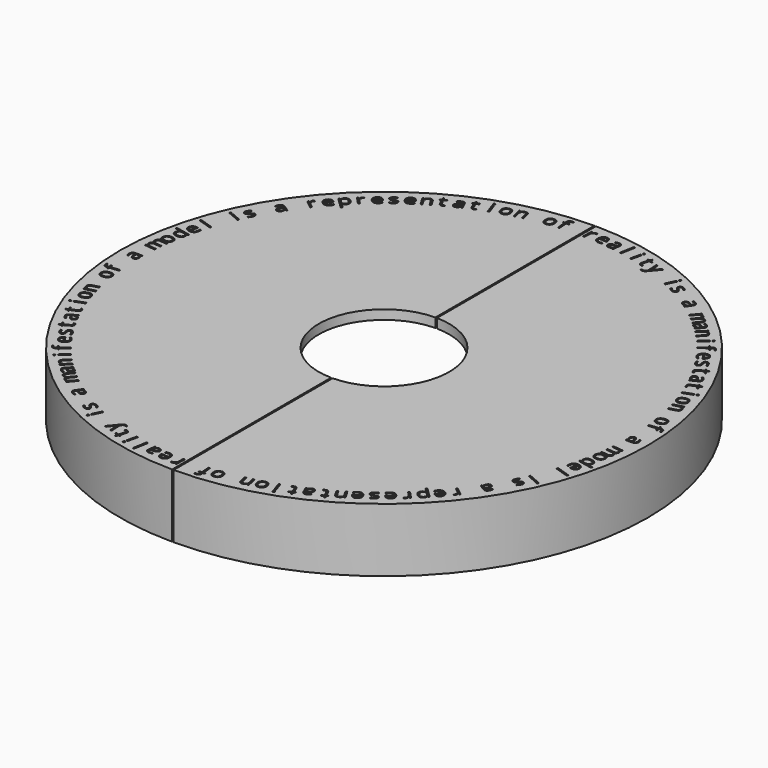
from build123d import *

# Parameters (mm, degrees)
F3_TEXT_SIZE = 6.25
F4_DEPTH     = 0.5
F5_W         = 0.5
F5_H         = 250
F6_DEPTH     = 20.5010001
F7_R         = 1.5
F8_DEPTH     = 1.5


# Not quite as in the source:
# - Text() gives the source's letters only with a copy of the font that has no kerning and outlines rounded to 1/6400 em; it was checked with that copy


with BuildPart() as f1:
    # F0 (on Front) → F1 (revolve)
    with BuildSketch(Plane.XZ):
        Polygon((-80.75, 17.5), (-21, 17.5), (-21, 20.5), (-80.75, 20.5), (-85, 20.5), (-85, 0), (-80.75, 0), align=None)
    revolve(axis=Axis((0, 0, 4.5), (0, 0, 1)))

    # F3 (on face) → F4 (cut)
    with BuildSketch(Plane.XY.offset(20.5)):
        with Locations(Location((78.75, 1.6875), (0, 0, -90))):
            Text('a', F3_TEXT_SIZE, font='Open Sans', text_align=(TextAlign.LEFT, TextAlign.BOTTOM))
        with Locations(Location((78.6262675544, -5.2563334208), (0, 0, -95.9016393443))):
            Text('m', F3_TEXT_SIZE, font='Open Sans', text_align=(TextAlign.LEFT, TextAlign.BOTTOM))
        with Locations(Location((78.106553141, -10.227138462), (0, 0, -98.8524590164))):
            Text('o', F3_TEXT_SIZE, font='Open Sans', text_align=(TextAlign.LEFT, TextAlign.BOTTOM))
        with Locations(Location((77.4631267415, -14.2984525124), (0, 0, -101.8032786885))):
            Text('d', F3_TEXT_SIZE, font='Open Sans', text_align=(TextAlign.LEFT, TextAlign.BOTTOM))
        with Locations(Location((76.6099263363, -18.3219724096), (0, 0, -104.7540983607))):
            Text('e', F3_TEXT_SIZE, font='Open Sans', text_align=(TextAlign.LEFT, TextAlign.BOTTOM))
        with Locations(Location((75.2404006968, -23.2587545179), (0, 0, -107.7049180328))):
            Text('l', F3_TEXT_SIZE, font='Open Sans', text_align=(TextAlign.LEFT, TextAlign.BOTTOM))
        with Locations(Location((72.4599055893, -30.8494022324), (0, 0, -113.606557377))):
            Text('i', F3_TEXT_SIZE, font='Open Sans', text_align=(TextAlign.LEFT, TextAlign.BOTTOM))
        with Locations(Location((71.1337657816, -33.8223559246), (0, 0, -116.5573770492))):
            Text('s', F3_TEXT_SIZE, font='Open Sans', text_align=(TextAlign.LEFT, TextAlign.BOTTOM))
        with Locations(Location((67.3530001634, -40.8409540196), (0, 0, -122.4590163934))):
            Text('a', F3_TEXT_SIZE, font='Open Sans', text_align=(TextAlign.LEFT, TextAlign.BOTTOM))
        with Locations(Location((12.0100738883, -77.8523354171), (0, 0, -172.6229508197))):
            Text('o', F3_TEXT_SIZE, font='Open Sans', text_align=(TextAlign.LEFT, TextAlign.BOTTOM))
        with Locations(Location((57.7536819392, -53.5710114351), (0, 0, -134.262295082))):
            Text('p', F3_TEXT_SIZE, font='Open Sans', text_align=(TextAlign.LEFT, TextAlign.BOTTOM))
        with Locations(Location((62.6394396742, -47.748504569), (0, 0, -128.3606557377))):
            Text('r', F3_TEXT_SIZE, font='Open Sans', text_align=(TextAlign.LEFT, TextAlign.BOTTOM))
        with Locations(Location((60.3349493388, -50.6405901873), (0, 0, -131.3114754098))):
            Text('e', F3_TEXT_SIZE, font='Open Sans', text_align=(TextAlign.LEFT, TextAlign.BOTTOM))
        with Locations(Location((54.5452272552, -56.8193389169), (0, 0, -137.2131147541))):
            Text('r', F3_TEXT_SIZE, font='Open Sans', text_align=(TextAlign.LEFT, TextAlign.BOTTOM))
        with Locations(Location((51.8231235243, -59.3223343642), (0, 0, -140.1639344262))):
            Text('e', F3_TEXT_SIZE, font='Open Sans', text_align=(TextAlign.LEFT, TextAlign.BOTTOM))
        with Locations(Location((48.5064692039, -62.0571256178), (0, 0, -143.1147540984))):
            Text('s', F3_TEXT_SIZE, font='Open Sans', text_align=(TextAlign.LEFT, TextAlign.BOTTOM))
        with Locations(Location((42.1423747186, -66.5513068223), (0, 0, -149.0163934426))):
            Text('n', F3_TEXT_SIZE, font='Open Sans', text_align=(TextAlign.LEFT, TextAlign.BOTTOM))
        with Locations(Location((45.4488729518, -64.3364238487), (0, 0, -146.0655737705))):
            Text('e', F3_TEXT_SIZE, font='Open Sans', text_align=(TextAlign.LEFT, TextAlign.BOTTOM))
        with Locations(Location((38.1053971012, -68.928074056), (0, 0, -151.9672131148))):
            Text('t', F3_TEXT_SIZE, font='Open Sans', text_align=(TextAlign.LEFT, TextAlign.BOTTOM))
        with Locations(Location((34.9116308373, -70.6086976833), (0, 0, -154.9180327869))):
            Text('a', F3_TEXT_SIZE, font='Open Sans', text_align=(TextAlign.LEFT, TextAlign.BOTTOM))
        with Locations(Location((30.8161804516, -72.4807816161), (0, 0, -157.868852459))):
            Text('t', F3_TEXT_SIZE, font='Open Sans', text_align=(TextAlign.LEFT, TextAlign.BOTTOM))
        with Locations(Location((26.5801571443, -74.1324408225), (0, 0, -160.8196721311))):
            Text('i', F3_TEXT_SIZE, font='Open Sans', text_align=(TextAlign.LEFT, TextAlign.BOTTOM))
        with Locations(Location((23.8477494353, -75.0767131111), (0, 0, -163.7704918033))):
            Text('o', F3_TEXT_SIZE, font='Open Sans', text_align=(TextAlign.LEFT, TextAlign.BOTTOM))
        with Locations(Location((7.4694002148, -78.4073935642), (0, 0, -175.5737704918))):
            Text('f', F3_TEXT_SIZE, font='Open Sans', text_align=(TextAlign.LEFT, TextAlign.BOTTOM))
        with Locations(Location((19.9070776726, -76.215250739), (0, 0, -166.7213114754))):
            Text('n', F3_TEXT_SIZE, font='Open Sans', text_align=(TextAlign.LEFT, TextAlign.BOTTOM))
        with Locations(Location((-0.5940416139, -78.7608164371), (0, 0, 178.5245901639))):
            Text('r', F3_TEXT_SIZE, font='Open Sans', text_align=(TextAlign.LEFT, TextAlign.BOTTOM))
        with Locations(Location((-4.2904331993, -78.6534657164), (0, 0, 175.5737704918))):
            Text('e', F3_TEXT_SIZE, font='Open Sans', text_align=(TextAlign.LEFT, TextAlign.BOTTOM))
        with Locations(Location((-8.4378384552, -78.3148328125), (0, 0, 172.6229508197))):
            Text('a', F3_TEXT_SIZE, font='Open Sans', text_align=(TextAlign.LEFT, TextAlign.BOTTOM))
        with Locations(Location((-13.4054905375, -77.603997205), (0, 0, 169.6721311475))):
            Text('l', F3_TEXT_SIZE, font='Open Sans', text_align=(TextAlign.LEFT, TextAlign.BOTTOM))
        with Locations(Location((-17.3589118661, -76.8166109311), (0, 0, 166.7213114754))):
            Text('i', F3_TEXT_SIZE, font='Open Sans', text_align=(TextAlign.LEFT, TextAlign.BOTTOM))
        with Locations(Location((-20.8186828661, -75.9584302433), (0, 0, 163.7704918033))):
            Text('t', F3_TEXT_SIZE, font='Open Sans', text_align=(TextAlign.LEFT, TextAlign.BOTTOM))
        with Locations(Location((-24.196797606, -74.9614969893), (0, 0, 160.8196721311))):
            Text('y', F3_TEXT_SIZE, font='Open Sans', text_align=(TextAlign.LEFT, TextAlign.BOTTOM))
        with Locations(Location((-32.704866046, -71.6415750317), (0, 0, 154.9180327869))):
            Text('i', F3_TEXT_SIZE, font='Open Sans', text_align=(TextAlign.LEFT, TextAlign.BOTTOM))
        with Locations(Location((-35.6426887742, -70.2393275275), (0, 0, 151.9672131148))):
            Text('s', F3_TEXT_SIZE, font='Open Sans', text_align=(TextAlign.LEFT, TextAlign.BOTTOM))
        with Locations(Location((-42.5616131492, -66.2791010982), (0, 0, 146.0655737705))):
            Text('a', F3_TEXT_SIZE, font='Open Sans', text_align=(TextAlign.LEFT, TextAlign.BOTTOM))
        with Locations(Location((-48.2536792635, -62.3000917183), (0, 0, 140.1639344262))):
            Text('m', F3_TEXT_SIZE, font='Open Sans', text_align=(TextAlign.LEFT, TextAlign.BOTTOM))
        with Locations(Location((-52.2543438823, -58.9397463659), (0, 0, 137.2131147541))):
            Text('a', F3_TEXT_SIZE, font='Open Sans', text_align=(TextAlign.LEFT, TextAlign.BOTTOM))
        with Locations(Location((-55.0924290561, -56.3016913367), (0, 0, 134.262295082))):
            Text('n', F3_TEXT_SIZE, font='Open Sans', text_align=(TextAlign.LEFT, TextAlign.BOTTOM))
        with Locations(Location((-58.6571701454, -52.5495949237), (0, 0, 131.3114754098))):
            Text('i', F3_TEXT_SIZE, font='Open Sans', text_align=(TextAlign.LEFT, TextAlign.BOTTOM))
        with Locations(Location((-60.8830663555, -49.9676248809), (0, 0, 128.3606557377))):
            Text('f', F3_TEXT_SIZE, font='Open Sans', text_align=(TextAlign.LEFT, TextAlign.BOTTOM))
        with Locations(Location((-63.1448805777, -47.0903338601), (0, 0, 125.4098360656))):
            Text('e', F3_TEXT_SIZE, font='Open Sans', text_align=(TextAlign.LEFT, TextAlign.BOTTOM))
        with Locations(Location((-65.6155510589, -43.5725125947), (0, 0, 122.4590163934))):
            Text('s', F3_TEXT_SIZE, font='Open Sans', text_align=(TextAlign.LEFT, TextAlign.BOTTOM))
        with Locations(Location((-67.9240876859, -39.8675180233), (0, 0, 119.5081967213))):
            Text('t', F3_TEXT_SIZE, font='Open Sans', text_align=(TextAlign.LEFT, TextAlign.BOTTOM))
        with Locations(Location((-69.6863869499, -36.7180831488), (0, 0, 116.5573770492))):
            Text('a', F3_TEXT_SIZE, font='Open Sans', text_align=(TextAlign.LEFT, TextAlign.BOTTOM))
        with Locations(Location((-71.663299529, -32.6721927934), (0, 0, 113.606557377))):
            Text('t', F3_TEXT_SIZE, font='Open Sans', text_align=(TextAlign.LEFT, TextAlign.BOTTOM))
        with Locations(Location((-73.423479919, -28.4801006441), (0, 0, 110.6557377049))):
            Text('i', F3_TEXT_SIZE, font='Open Sans', text_align=(TextAlign.LEFT, TextAlign.BOTTOM))
        with Locations(Location((-74.4377929484, -25.7729118584), (0, 0, 107.7049180328))):
            Text('o', F3_TEXT_SIZE, font='Open Sans', text_align=(TextAlign.LEFT, TextAlign.BOTTOM))
        with Locations(Location((-75.6774171905, -21.8628615249), (0, 0, 104.7540983607))):
            Text('n', F3_TEXT_SIZE, font='Open Sans', text_align=(TextAlign.LEFT, TextAlign.BOTTOM))
        with Locations(Location((-77.5172904933, -14.0106273688), (0, 0, 98.8524590164))):
            Text('o', F3_TEXT_SIZE, font='Open Sans', text_align=(TextAlign.LEFT, TextAlign.BOTTOM))
        with Locations(Location((-78.1890774943, -9.4857506654), (0, 0, 95.9016393443))):
            Text('f', F3_TEXT_SIZE, font='Open Sans', text_align=(TextAlign.LEFT, TextAlign.BOTTOM))
        with Locations(Location((-78.75, -1.6875), (0, 0, 90))):
            Text('a', F3_TEXT_SIZE, font='Open Sans', text_align=(TextAlign.LEFT, TextAlign.BOTTOM))
        with Locations(Location((-78.6262675544, 5.2563334208), (0, 0, 84.0983606557))):
            Text('m', F3_TEXT_SIZE, font='Open Sans', text_align=(TextAlign.LEFT, TextAlign.BOTTOM))
        with Locations(Location((-78.106553141, 10.227138462), (0, 0, 81.1475409836))):
            Text('o', F3_TEXT_SIZE, font='Open Sans', text_align=(TextAlign.LEFT, TextAlign.BOTTOM))
        with Locations(Location((-77.4631267415, 14.2984525124), (0, 0, 78.1967213115))):
            Text('d', F3_TEXT_SIZE, font='Open Sans', text_align=(TextAlign.LEFT, TextAlign.BOTTOM))
        with Locations(Location((-76.6099263363, 18.3219724096), (0, 0, 75.2459016393))):
            Text('e', F3_TEXT_SIZE, font='Open Sans', text_align=(TextAlign.LEFT, TextAlign.BOTTOM))
        with Locations(Location((-75.2404006968, 23.2587545179), (0, 0, 72.2950819672))):
            Text('l', F3_TEXT_SIZE, font='Open Sans', text_align=(TextAlign.LEFT, TextAlign.BOTTOM))
        with Locations(Location((-72.4599055893, 30.8494022324), (0, 0, 66.393442623))):
            Text('i', F3_TEXT_SIZE, font='Open Sans', text_align=(TextAlign.LEFT, TextAlign.BOTTOM))
        with Locations(Location((-71.1337657816, 33.8223559246), (0, 0, 63.4426229508))):
            Text('s', F3_TEXT_SIZE, font='Open Sans', text_align=(TextAlign.LEFT, TextAlign.BOTTOM))
        with Locations(Location((-67.3530001634, 40.8409540196), (0, 0, 57.5409836066))):
            Text('a', F3_TEXT_SIZE, font='Open Sans', text_align=(TextAlign.LEFT, TextAlign.BOTTOM))
        with Locations(Location((-62.6394396742, 47.748504569), (0, 0, 51.6393442623))):
            Text('r', F3_TEXT_SIZE, font='Open Sans', text_align=(TextAlign.LEFT, TextAlign.BOTTOM))
        with Locations(Location((-60.3349493388, 50.6405901873), (0, 0, 48.6885245902))):
            Text('e', F3_TEXT_SIZE, font='Open Sans', text_align=(TextAlign.LEFT, TextAlign.BOTTOM))
        with Locations(Location((-57.7536819392, 53.5710114351), (0, 0, 45.737704918))):
            Text('p', F3_TEXT_SIZE, font='Open Sans', text_align=(TextAlign.LEFT, TextAlign.BOTTOM))
        with Locations(Location((-54.5452272552, 56.8193389169), (0, 0, 42.7868852459))):
            Text('r', F3_TEXT_SIZE, font='Open Sans', text_align=(TextAlign.LEFT, TextAlign.BOTTOM))
        with Locations(Location((-51.8231235243, 59.3223343642), (0, 0, 39.8360655738))):
            Text('e', F3_TEXT_SIZE, font='Open Sans', text_align=(TextAlign.LEFT, TextAlign.BOTTOM))
        with Locations(Location((-48.5064692039, 62.0571256178), (0, 0, 36.8852459016))):
            Text('s', F3_TEXT_SIZE, font='Open Sans', text_align=(TextAlign.LEFT, TextAlign.BOTTOM))
        with Locations(Location((-45.4488729518, 64.3364238487), (0, 0, 33.9344262295))):
            Text('e', F3_TEXT_SIZE, font='Open Sans', text_align=(TextAlign.LEFT, TextAlign.BOTTOM))
        with Locations(Location((-42.1423747186, 66.5513068223), (0, 0, 30.9836065574))):
            Text('n', F3_TEXT_SIZE, font='Open Sans', text_align=(TextAlign.LEFT, TextAlign.BOTTOM))
        with Locations(Location((-38.1053971012, 68.928074056), (0, 0, 28.0327868852))):
            Text('t', F3_TEXT_SIZE, font='Open Sans', text_align=(TextAlign.LEFT, TextAlign.BOTTOM))
        with Locations(Location((-34.9116308373, 70.6086976833), (0, 0, 25.0819672131))):
            Text('a', F3_TEXT_SIZE, font='Open Sans', text_align=(TextAlign.LEFT, TextAlign.BOTTOM))
        with Locations(Location((-30.8161804516, 72.4807816161), (0, 0, 22.131147541))):
            Text('t', F3_TEXT_SIZE, font='Open Sans', text_align=(TextAlign.LEFT, TextAlign.BOTTOM))
        with Locations(Location((-26.5801571443, 74.1324408225), (0, 0, 19.1803278689))):
            Text('i', F3_TEXT_SIZE, font='Open Sans', text_align=(TextAlign.LEFT, TextAlign.BOTTOM))
        with Locations(Location((-23.8477494353, 75.0767131111), (0, 0, 16.2295081967))):
            Text('o', F3_TEXT_SIZE, font='Open Sans', text_align=(TextAlign.LEFT, TextAlign.BOTTOM))
        with Locations(Location((-19.9070776726, 76.215250739), (0, 0, 13.2786885246))):
            Text('n', F3_TEXT_SIZE, font='Open Sans', text_align=(TextAlign.LEFT, TextAlign.BOTTOM))
        with Locations(Location((-12.0100738883, 77.8523354171), (0, 0, 7.3770491803))):
            Text('o', F3_TEXT_SIZE, font='Open Sans', text_align=(TextAlign.LEFT, TextAlign.BOTTOM))
        with Locations(Location((-7.4694002148, 78.4073935642), (0, 0, 4.4262295082))):
            Text('f', F3_TEXT_SIZE, font='Open Sans', text_align=(TextAlign.LEFT, TextAlign.BOTTOM))
        with Locations(Location((0.5940416139, 78.7608164371), (0, 0, -1.4754098361))):
            Text('r', F3_TEXT_SIZE, font='Open Sans', text_align=(TextAlign.LEFT, TextAlign.BOTTOM))
        with Locations(Location((4.2904331993, 78.6534657164), (0, 0, -4.4262295082))):
            Text('e', F3_TEXT_SIZE, font='Open Sans', text_align=(TextAlign.LEFT, TextAlign.BOTTOM))
        with Locations(Location((8.4378384552, 78.3148328125), (0, 0, -7.3770491803))):
            Text('a', F3_TEXT_SIZE, font='Open Sans', text_align=(TextAlign.LEFT, TextAlign.BOTTOM))
        with Locations(Location((13.4054905375, 77.603997205), (0, 0, -10.3278688525))):
            Text('l', F3_TEXT_SIZE, font='Open Sans', text_align=(TextAlign.LEFT, TextAlign.BOTTOM))
        with Locations(Location((17.3589118661, 76.8166109311), (0, 0, -13.2786885246))):
            Text('i', F3_TEXT_SIZE, font='Open Sans', text_align=(TextAlign.LEFT, TextAlign.BOTTOM))
        with Locations(Location((20.8186828661, 75.9584302433), (0, 0, -16.2295081967))):
            Text('t', F3_TEXT_SIZE, font='Open Sans', text_align=(TextAlign.LEFT, TextAlign.BOTTOM))
        with Locations(Location((24.196797606, 74.9614969893), (0, 0, -19.1803278689))):
            Text('y', F3_TEXT_SIZE, font='Open Sans', text_align=(TextAlign.LEFT, TextAlign.BOTTOM))
        with Locations(Location((32.704866046, 71.6415750317), (0, 0, -25.0819672131))):
            Text('i', F3_TEXT_SIZE, font='Open Sans', text_align=(TextAlign.LEFT, TextAlign.BOTTOM))
        with Locations(Location((35.6426887742, 70.2393275275), (0, 0, -28.0327868852))):
            Text('s', F3_TEXT_SIZE, font='Open Sans', text_align=(TextAlign.LEFT, TextAlign.BOTTOM))
        with Locations(Location((42.5616131492, 66.2791010982), (0, 0, -33.9344262295))):
            Text('a', F3_TEXT_SIZE, font='Open Sans', text_align=(TextAlign.LEFT, TextAlign.BOTTOM))
        with Locations(Location((48.2536792635, 62.3000917183), (0, 0, -39.8360655738))):
            Text('m', F3_TEXT_SIZE, font='Open Sans', text_align=(TextAlign.LEFT, TextAlign.BOTTOM))
        with Locations(Location((52.2543438823, 58.9397463659), (0, 0, -42.7868852459))):
            Text('a', F3_TEXT_SIZE, font='Open Sans', text_align=(TextAlign.LEFT, TextAlign.BOTTOM))
        with Locations(Location((55.0924290561, 56.3016913367), (0, 0, -45.737704918))):
            Text('n', F3_TEXT_SIZE, font='Open Sans', text_align=(TextAlign.LEFT, TextAlign.BOTTOM))
        with Locations(Location((58.6571701454, 52.5495949237), (0, 0, -48.6885245902))):
            Text('i', F3_TEXT_SIZE, font='Open Sans', text_align=(TextAlign.LEFT, TextAlign.BOTTOM))
        with Locations(Location((60.8830663555, 49.9676248809), (0, 0, -51.6393442623))):
            Text('f', F3_TEXT_SIZE, font='Open Sans', text_align=(TextAlign.LEFT, TextAlign.BOTTOM))
        with Locations(Location((63.1448805777, 47.0903338601), (0, 0, -54.5901639344))):
            Text('e', F3_TEXT_SIZE, font='Open Sans', text_align=(TextAlign.LEFT, TextAlign.BOTTOM))
        with Locations(Location((65.6155510589, 43.5725125947), (0, 0, -57.5409836066))):
            Text('s', F3_TEXT_SIZE, font='Open Sans', text_align=(TextAlign.LEFT, TextAlign.BOTTOM))
        with Locations(Location((67.9240876859, 39.8675180233), (0, 0, -60.4918032787))):
            Text('t', F3_TEXT_SIZE, font='Open Sans', text_align=(TextAlign.LEFT, TextAlign.BOTTOM))
        with Locations(Location((69.6863869499, 36.7180831488), (0, 0, -63.4426229508))):
            Text('a', F3_TEXT_SIZE, font='Open Sans', text_align=(TextAlign.LEFT, TextAlign.BOTTOM))
        with Locations(Location((71.663299529, 32.6721927934), (0, 0, -66.393442623))):
            Text('t', F3_TEXT_SIZE, font='Open Sans', text_align=(TextAlign.LEFT, TextAlign.BOTTOM))
        with Locations(Location((73.423479919, 28.4801006441), (0, 0, -69.3442622951))):
            Text('i', F3_TEXT_SIZE, font='Open Sans', text_align=(TextAlign.LEFT, TextAlign.BOTTOM))
        with Locations(Location((74.4377929484, 25.7729118584), (0, 0, -72.2950819672))):
            Text('o', F3_TEXT_SIZE, font='Open Sans', text_align=(TextAlign.LEFT, TextAlign.BOTTOM))
        with Locations(Location((75.6774171905, 21.8628615249), (0, 0, -75.2459016393))):
            Text('n', F3_TEXT_SIZE, font='Open Sans', text_align=(TextAlign.LEFT, TextAlign.BOTTOM))
        with Locations(Location((77.5172904933, 14.0106273688), (0, 0, -81.1475409836))):
            Text('o', F3_TEXT_SIZE, font='Open Sans', text_align=(TextAlign.LEFT, TextAlign.BOTTOM))
        with Locations(Location((78.1890774943, 9.4857506654), (0, 0, -84.0983606557))):
            Text('f', F3_TEXT_SIZE, font='Open Sans', text_align=(TextAlign.LEFT, TextAlign.BOTTOM))
    extrude(amount=-F4_DEPTH, mode=Mode.SUBTRACT)

    # F5 (on Top) → F6 (cut, through all)
    with BuildSketch(Plane.XY):
        Rectangle(F5_W, F5_H)
    extrude(amount=F6_DEPTH, mode=Mode.SUBTRACT)

    # F7 (on Right) → F8 (cut, symmetric)
    with BuildSketch(Plane.YZ):
        with Locations((-82.8746323521, 17.4853662029)):
            Circle(F7_R)
        with Locations((82.8746323521, 17.4853662029)):
            Circle(F7_R)
    extrude(amount=F8_DEPTH, both=True, mode=Mode.SUBTRACT)


solid = f1.part
